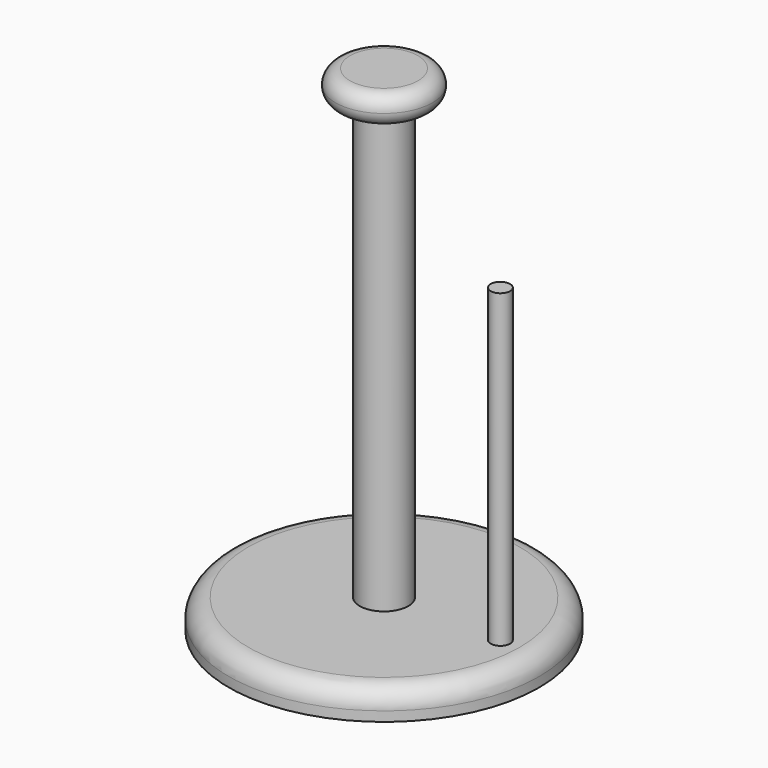
from build123d import *

# Parameters (mm, degrees)
F0_R      = 101.6
F1_DEPTH  = 19.05
F2_R      = 12.7
F3_R      = 15.875
F4_DEPTH  = 285.75
F3_R_2    = 6.35
F5_DEPTH  = 203.2
F6_R      = 31.75
F7_DEPTH  = 19.05
F8_R      = 9.52499
F9_D      = 6.7564
F9_DEPTH  = 25.4
F9_TIP    = 2.0298273432
F10_D     = 6.7564
F10_DEPTH = 12.7
F10_TIP   = 2.0298273432


# Not quite as in the source:
# - a fillet or chamfer is up to 0.001 mm smaller than in the source, because OpenCascade refuses the exact size


with BuildPart() as f1:
    # F0 (on Top) → F1 (new body)
    with BuildSketch(Plane.XY):
        Circle(F0_R)
    extrude(amount=F1_DEPTH)

    # F2
    f2_edges = [f1.edges().sort_by_distance(p)[0] for p in [
        (-101.6, 0, 19.05),
    ]]
    fillet(f2_edges, radius=F2_R)


with BuildPart() as f4:
    # F3 (on face) → F4 (new body)
    with BuildSketch(Plane.XY.offset(19.05)):
        Circle(F3_R)
    extrude(amount=F4_DEPTH)

    # F9
    with Locations(Plane.XY.offset(304.8)):
        with Locations((0, 0)):
            Hole(F9_D / 2, depth=F9_DEPTH)
            with Locations((0, 0, -(F9_DEPTH + F9_TIP / 2))):  # 118° drill point
                Cone(0, F9_D / 2, F9_TIP, mode=Mode.SUBTRACT)


with BuildPart() as f5:
    # F3 (on face) → F5 (new body)
    with BuildSketch(Plane.XY.offset(19.05)):
        with Locations((76.2, 0)):
            Circle(F3_R_2)
    extrude(amount=F5_DEPTH)


with BuildPart() as f7:
    # F6 (on face) → F7 (new body)
    with BuildSketch(Plane.XY.offset(304.8)):
        Circle(F6_R)
    extrude(amount=F7_DEPTH)

    # F8 (radius 9.525 in the source; OpenCascade refuses exactly that, so slightly less here)
    f8_edges = [f7.edges().sort_by_distance(p)[0] for p in [
        (-31.75, 0, 323.85),
        (-31.75, 0, 304.8),
    ]]
    fillet(f8_edges, radius=F8_R)

    # F10
    with Locations(Plane(origin=(0, 0, 304.8), x_dir=(1, 0, 0), z_dir=(0, 0, -1))):
        with Locations((0, 0)):
            Hole(F10_D / 2, depth=F10_DEPTH)
            with Locations((0, 0, -(F10_DEPTH + F10_TIP / 2))):  # 118° drill point
                Cone(0, F10_D / 2, F10_TIP, mode=Mode.SUBTRACT)


solid = Compound([f1.part, f4.part, f5.part, f7.part])
